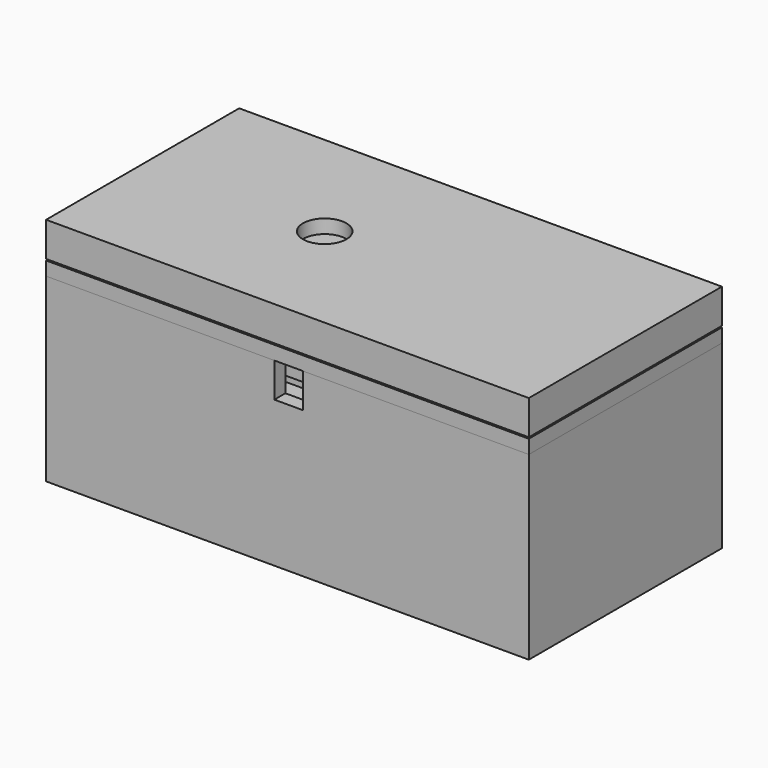
from build123d import *

# Parameters (mm, degrees)
F0_W      = 70
F0_H      = 35
F1_DEPTH  = 2
F2_W      = 70
F2_H      = 35
F2_W_2    = 66
F2_H_2    = 31
F3_DEPTH  = 24.2
F5_DEPTH  = 15.5
F6_W      = 70
F6_H      = 35
F7_DEPTH  = 2
F8_W      = 65.2
F8_H      = 30.2
F8_W_2    = 61.2
F8_H_2    = 26.2
F9_DEPTH  = 3
F11_DEPTH = 25
F13_DEPTH = 5
F14_R     = 1
F15_DEPTH = 3
F17_W     = 70
F17_H     = 35
F18_DEPTH = 2
F19_W     = 70
F19_H     = 35
F19_W_2   = 66
F19_H_2   = 31
F20_DEPTH = 3
F21_R     = 3.15
F22_DEPTH = 2
F23_R     = 1.5
F24_DEPTH = 6
F25_R     = 1.6
F26_DEPTH = 2


with BuildPart() as f1:
    # F0 (on Top) → F1 (new body)
    with BuildSketch(Plane.XY):
        Rectangle(F0_W, F0_H)
    extrude(amount=F1_DEPTH)

    # F2 (on face) → F3 (join)
    with BuildSketch(Plane.XY.offset(2)):
        Rectangle(F2_W, F2_H)
        Rectangle(F2_W_2, F2_H_2, mode=Mode.SUBTRACT)
    extrude(amount=F3_DEPTH)

    # F4 (on face) → F5 (join)
    with BuildSketch(Plane.XY.offset(2)):
        Polygon((3.7, 6.5), (28.3, 6.5), (28.3, -6.5), (3.7, -6.5), (3.7, -2), (1.7, -2), (1.7, -8.5), (30.3, -8.5), (30.3, 8.5), (1.7, 8.5), (1.7, 2), (3.7, 2), align=None)
    extrude(amount=F5_DEPTH)

    # F12 (on face) → F13 (cut)
    with BuildSketch(Plane(origin=(0, 0, 26.2), x_dir=(1, 0, 0), z_dir=(0, 0, -1))):
        Polygon((-1.899776631, 17.714696005), (-1.899776631, 15.3786540031), (-1.899776631, 15.1450503618), (2.227232093, 15.1450503618), (2.227232093, 17.714696005), align=None)
    extrude(amount=F13_DEPTH, mode=Mode.SUBTRACT)


with BuildPart() as f7:
    # F6 (on face) → F7 (new body)
    with BuildSketch(Plane.XY.offset(26.2)):
        Rectangle(F6_W, F6_H)
    extrude(amount=F7_DEPTH)

    # F8 (on face) → F9 (join)
    with BuildSketch(Plane(origin=(0, 0, 26.2), x_dir=(1, 0, 0), z_dir=(0, 0, -1))):
        Rectangle(F8_W, F8_H)
        Rectangle(F8_W_2, F8_H_2, mode=Mode.SUBTRACT)
    extrude(amount=F9_DEPTH)

    # F10 (on face) → F11 (cut)
    with BuildSketch(Plane(origin=(0, 0, 26.2), x_dir=(1, 0, 0), z_dir=(0, 0, -1))):
        with BuildLine():
            ThreePointArc((15.7376033058, -3.3503810132), (16.4913728942, -1.75), (16.75, 0))
            ThreePointArc((16.75, 0), (16.4913728942, 1.75), (15.7376033058, 3.3503810132))
            ThreePointArc((15.7376033058, 3.3503810132), (13.25, 0), (15.7376033058, -3.3503810132))
        make_face()
        with BuildLine():
            ThreePointArc((15.7376033058, 3.3503810132), (16.4913728942, 1.75), (16.75, 0))
            ThreePointArc((16.75, 0), (16.4913728942, -1.75), (15.7376033058, -3.3503810132))
            ThreePointArc((15.7376033058, -3.3503810132), (18.8364577123, -2.8101057302), (20.25, 0))
            ThreePointArc((20.25, 0), (18.8364577123, 2.8101057302), (15.7376033058, 3.3503810132))
        make_face()
        with BuildLine():
            ThreePointArc((15.7376033058, -3.3503810132), (13.25, 0), (15.7376033058, 3.3503810132))
            ThreePointArc((15.7376033058, 3.3503810132), (4.65, 0), (15.7376033058, -3.3503810132))
        make_face()
    extrude(amount=-F11_DEPTH, mode=Mode.SUBTRACT)

    # F14 (on face) → F15 (cut)
    with BuildSketch(Plane.XY.offset(28.2)):
        with Locations((-8.6, 0)):
            Circle(F14_R)
    extrude(amount=-F15_DEPTH, mode=Mode.SUBTRACT)

    # F25 (on face) → F26 (cut)
    with BuildSketch(Plane.XY.offset(28.2)):
        with Locations((-24.5572296758, 10.8354858681)):
            Circle(F25_R)
        with Locations((-24.0306204174, -9.4215996393)):
            Circle(F25_R)
        with Locations((26.737968057, -10.1487416467)):
            Circle(F25_R)
    extrude(amount=-F26_DEPTH, mode=Mode.SUBTRACT)


with BuildPart() as f18:
    # F17 (on offset) → F18 (new body)
    with BuildSketch(Plane.XY.offset(31.4)):
        Rectangle(F17_W, F17_H)
    extrude(amount=F18_DEPTH)

    # F19 (on offset) → F20 (join)
    with BuildSketch(Plane.XY.offset(31.4)):
        Rectangle(F19_W, F19_H)
        Rectangle(F19_W_2, F19_H_2, mode=Mode.SUBTRACT)
    extrude(amount=-F20_DEPTH)

    # F21 (on face) → F22 (cut)
    with BuildSketch(Plane.XY.offset(33.4)):
        with Locations((-8.6, 0)):
            Circle(F21_R)
    extrude(amount=-F22_DEPTH, mode=Mode.SUBTRACT)

    # F23 (on offset) → F24 (join)
    with BuildSketch(Plane.XY.offset(31.4)):
        with Locations((-24.5937554311, 10.8404249086)):
            Circle(F23_R)
        with Locations((-24.0737235235, -9.4408045343)):
            Circle(F23_R)
        with Locations((26.7853572811, -10.1688477976)):
            Circle(F23_R)
    extrude(amount=-F24_DEPTH)


solid = Compound([f1.part, f7.part, f18.part])
